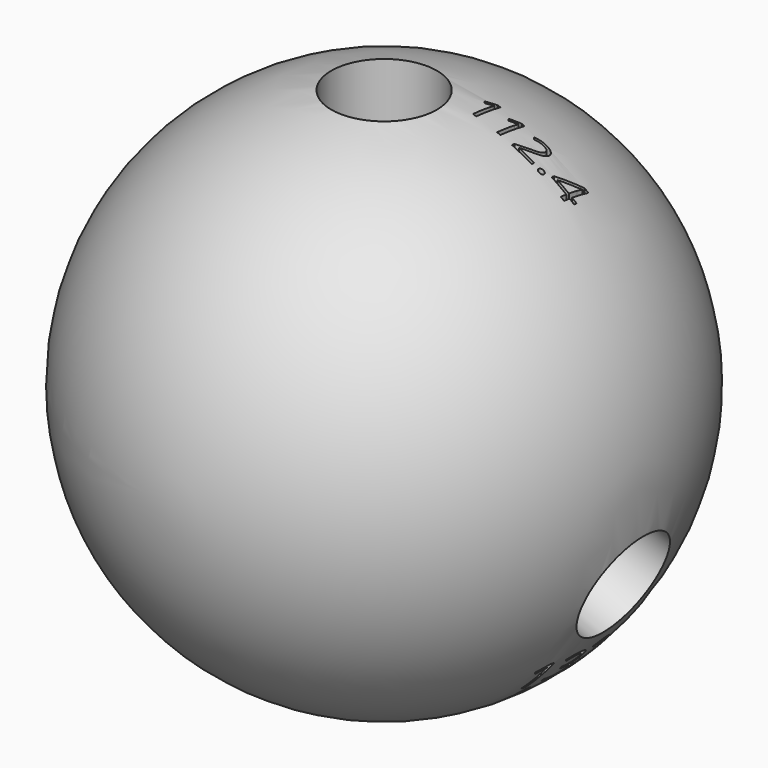
from build123d import *

# Parameters (mm, degrees)
F4_R          = 3.175
F5_DEPTH      = 25.4
F7_TEXT_SIZE  = 2.5403220206
F8_DEPTH      = 7.8994
F9_ANGLE      = 112.4
F10_ANGLE     = 132.7
F12_TEXT_SIZE = 3.3532269299
F13_DEPTH     = 6.2484
F15_TEXT_SIZE = 2.1365571431
F16_DEPTH     = 5.7912


# Not quite as in the source:
# - Text() gives the source's letters only with a copy of the font that has no kerning and outlines rounded to 1/6400 em; it was checked with that copy


with BuildPart() as f2:
    # F1 (on Top) → F2 (revolve)
    with BuildSketch(Plane.XY):
        with BuildLine():
            Line((0, -15.875), (0, 15.875))
            ThreePointArc((0, 15.875), (-15.875, 0), (0, -15.875))
        make_face()
    revolve(axis=Axis((0, 0, 0), (0, -1, 0)))

    # F7 (on offset) → F8 (cut)
    with BuildSketch(Plane.XY.offset(17.0942)):
        with Locations((3.6763319804, 1.2244633399)):
            Text('112.4', F7_TEXT_SIZE, font='Open Sans', text_align=(TextAlign.LEFT, TextAlign.BOTTOM))
    extrude(amount=-F8_DEPTH, mode=Mode.SUBTRACT)

    # F12 (on offset) → F13 (cut)
    with BuildSketch(Plane(origin=(17.6126019403, 0, -7.2593906695), x_dir=(0, 1, 0), z_dir=(0.9245460336, 0, -0.3810703764))):
        with Locations((-3.7312244531, -6.6942567937)):
            Text('132.7', F12_TEXT_SIZE, font='Open Sans', text_align=(TextAlign.LEFT, TextAlign.BOTTOM))
    extrude(amount=-F13_DEPTH, mode=Mode.SUBTRACT)

    # F15 (on offset) → F16 (cut)
    with BuildSketch(Plane(origin=(-17.2791884723, 0, -8.0207322447), x_dir=(0, -1, 0), z_dir=(-0.9070440143, 0, -0.4210358134))):
        with Locations((-3.7359406706, 3.904532874)):
            Text('114.9', F15_TEXT_SIZE, font='Open Sans', text_align=(TextAlign.LEFT, TextAlign.BOTTOM))
    extrude(amount=-F16_DEPTH, mode=Mode.SUBTRACT)


with BuildPart() as f5:
    # F4 (on offset) → F5 (new body)
    with BuildSketch(Plane.XY.offset(6.35)):
        Circle(F4_R)
    extrude(amount=F5_DEPTH)


with BuildPart() as f9_1:
    # F9: copy of F5
    add(f5.part.rotate(Axis((0, 33.2760475576, 0), (0, 1, 0)), F9_ANGLE))


with BuildPart() as f10_1:
    # F10: copy of F9_1
    add(f9_1.part.rotate(Axis((0, 33.2760475576, 0), (0, 1, 0)), F10_ANGLE))


with BuildPart() as f2_1:
    add(f2.part)

    # F17: cut F5, F10_1, F9_1
    add(f5.part, mode=Mode.SUBTRACT)
    add(f10_1.part, mode=Mode.SUBTRACT)
    add(f9_1.part, mode=Mode.SUBTRACT)


solid = f2_1.part
